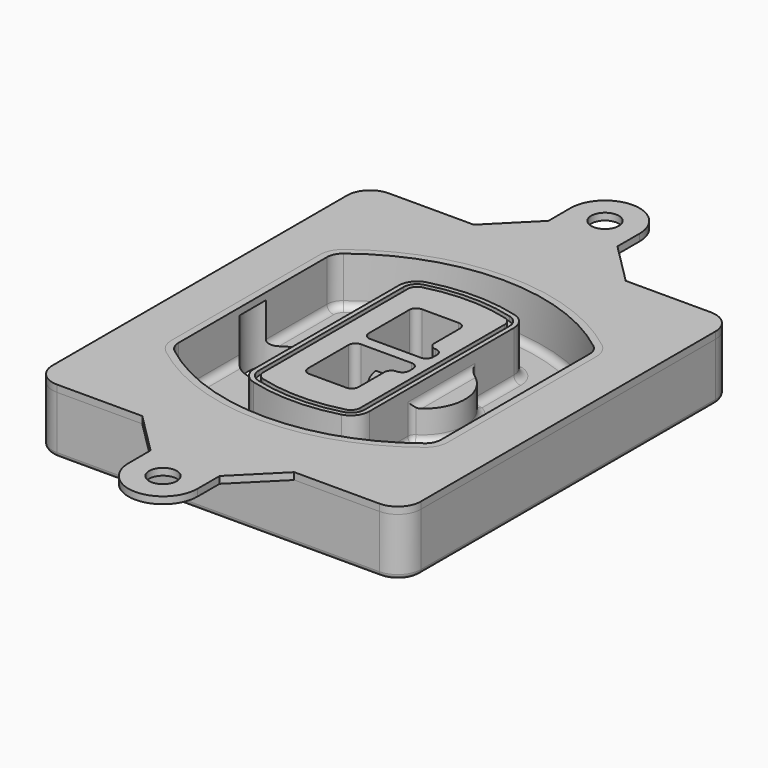
from build123d import *

# Parameters (mm, degrees)
F0_R      = 4
F1_DEPTH  = 25
F2_DEPTH  = 3
F3_DEPTH  = 18
F5_DEPTH  = 21
F6_DEPTH  = 2
F8_DEPTH  = 20
F9_DEPTH  = 16
F10_DEPTH = 25
F7_R      = 6
F7_R_2    = 4
F11_DEPTH = 6
F13_DEPTH = 9
F14_R     = 3
F16_R     = 2
F15_R     = 6
F17_DEPTH = 3


# Not quite as in the source:
# - a feature names something its author has since deleted; it is built from what else it names


with BuildPart() as f1:
    # F0 (on Top) → F1 (new body)
    with BuildSketch(Plane.XY):
        with BuildLine():
            ThreePointArc((-80, -80), (-77.0710678119, -87.0710678119), (-70, -90))
            Line((-70, -90), (70, -90))
            ThreePointArc((70, -90), (77.0710678119, -87.0710678119), (80, -80))
            Line((80, -80), (80, 80))
            ThreePointArc((80, 80), (77.0710678119, 87.0710678119), (70, 90))
            Line((70, 90), (-70, 90))
            ThreePointArc((-70, 90), (-77.0710678119, 87.0710678119), (-80, 80))
            Line((-80, 80), (-80, -80))
        make_face()
        with Locations((-60, -67.5)):
            Circle(F0_R, mode=Mode.SUBTRACT)
        with Locations((60, -67.5)):
            Circle(F0_R, mode=Mode.SUBTRACT)
        with Locations((-60, 67.5)):
            Circle(F0_R, mode=Mode.SUBTRACT)
        with BuildLine():
            ThreePointArc((-64, 40.2934422872), (-62.5820384798, 46.4328484224), (-58.6153846154, 51.3286200352))
            ThreePointArc((-58.6153846154, 51.3286200352), (0, 71.5), (58.6153846154, 51.3286200352))
            ThreePointArc((58.6153846154, 51.3286200352), (62.5820384798, 46.4328484224), (64, 40.2934422872))
            Line((64, 40.2934422872), (64, -40.2934422872))
            ThreePointArc((64, -40.2934422872), (62.5820384798, -46.4328484224), (58.6153846154, -51.3286200352))
            ThreePointArc((58.6153846154, -51.3286200352), (0, -71.5), (-58.6153846154, -51.3286200352))
            ThreePointArc((-58.6153846154, -51.3286200352), (-62.5820384798, -46.4328484224), (-64, -40.2934422872))
            Line((-64, -40.2934422872), (-64, 40.2934422872))
        make_face(mode=Mode.SUBTRACT)
        with Locations((60, 67.5)):
            Circle(F0_R, mode=Mode.SUBTRACT)
        with BuildLine():
            ThreePointArc((58.6153846154, 51.3286200352), (0, 71.5), (-58.6153846154, 51.3286200352))
            ThreePointArc((-58.6153846154, 51.3286200352), (-62.5820384798, 46.4328484224), (-64, 40.2934422872))
            Line((-64, 40.2934422872), (-64, -40.2934422872))
            ThreePointArc((-64, -40.2934422872), (-62.5820384798, -46.4328484224), (-58.6153846154, -51.3286200352))
            ThreePointArc((-58.6153846154, -51.3286200352), (0, -71.5), (58.6153846154, -51.3286200352))
            ThreePointArc((58.6153846154, -51.3286200352), (62.5820384798, -46.4328484224), (64, -40.2934422872))
            Line((64, -40.2934422872), (64, 40.2934422872))
            ThreePointArc((64, 40.2934422872), (62.5820384798, 46.4328484224), (58.6153846154, 51.3286200352))
        make_face()
        with BuildLine():
            Line((-60, -40.2934422872), (-60, 40.2934422872))
            ThreePointArc((-60, 40.2934422872), (-58.9871703427, 44.6787323838), (-56.1538461538, 48.1757121072))
            ThreePointArc((-56.1538461538, 48.1757121072), (0, 67.5), (56.1538461538, 48.1757121072))
            ThreePointArc((56.1538461538, 48.1757121072), (58.9871703427, 44.6787323838), (60, 40.2934422872))
            Line((60, 40.2934422872), (60, -40.2934422872))
            ThreePointArc((60, -40.2934422872), (58.9871703427, -44.6787323838), (56.1538461538, -48.1757121072))
            ThreePointArc((56.1538461538, -48.1757121072), (0, -67.5), (-56.1538461538, -48.1757121072))
            ThreePointArc((-56.1538461538, -48.1757121072), (-58.9871703427, -44.6787323838), (-60, -40.2934422872))
        make_face(mode=Mode.SUBTRACT)
        with BuildLine():
            ThreePointArc((-56.1538461538, 48.1757121072), (-58.9871703427, 44.6787323838), (-60, 40.2934422872))
            Line((-60, 40.2934422872), (-60, -40.2934422872))
            ThreePointArc((-60, -40.2934422872), (-58.9871703427, -44.6787323838), (-56.1538461538, -48.1757121072))
            ThreePointArc((-56.1538461538, -48.1757121072), (0, -67.5), (56.1538461538, -48.1757121072))
            ThreePointArc((56.1538461538, -48.1757121072), (58.9871703427, -44.6787323838), (60, -40.2934422872))
            Line((60, -40.2934422872), (60, 40.2934422872))
            ThreePointArc((60, 40.2934422872), (58.9871703427, 44.6787323838), (56.1538461538, 48.1757121072))
            ThreePointArc((56.1538461538, 48.1757121072), (0, 67.5), (-56.1538461538, 48.1757121072))
        make_face()
        with BuildLine():
            ThreePointArc((54.3076923077, 45.8110311612), (56.2910192399, 43.3631453548), (57, 40.2934422872))
            Line((57, 40.2934422872), (57, -40.2934422872))
            ThreePointArc((57, -40.2934422872), (56.2910192399, -43.3631453548), (54.3076923077, -45.8110311612))
            ThreePointArc((54.3076923077, -45.8110311612), (0, -64.5), (-54.3076923077, -45.8110311612))
            ThreePointArc((-54.3076923077, -45.8110311612), (-56.2910192399, -43.3631453548), (-57, -40.2934422872))
            Line((-57, -40.2934422872), (-57, 40.2934422872))
            ThreePointArc((-57, 40.2934422872), (-56.2910192399, 43.3631453548), (-54.3076923077, 45.8110311612))
            ThreePointArc((-54.3076923077, 45.8110311612), (0, 64.5), (54.3076923077, 45.8110311612))
        make_face(mode=Mode.SUBTRACT)
        with BuildLine():
            Line((57, -40.2934422872), (57, 40.2934422872))
            ThreePointArc((57, 40.2934422872), (56.2910192399, 43.3631453548), (54.3076923077, 45.8110311612))
            ThreePointArc((54.3076923077, 45.8110311612), (0, 64.5), (-54.3076923077, 45.8110311612))
            ThreePointArc((-54.3076923077, 45.8110311612), (-56.2910192399, 43.3631453548), (-57, 40.2934422872))
            Line((-57, 40.2934422872), (-57, -40.2934422872))
            ThreePointArc((-57, -40.2934422872), (-56.2910192399, -43.3631453548), (-54.3076923077, -45.8110311612))
            ThreePointArc((-54.3076923077, -45.8110311612), (0, -64.5), (54.3076923077, -45.8110311612))
            ThreePointArc((54.3076923077, -45.8110311612), (56.2910192399, -43.3631453548), (57, -40.2934422872))
        make_face()
    extrude(amount=-F1_DEPTH)

    # F0 (on Top) → F2 (join)
    with BuildSketch(Plane.XY):
        with BuildLine():
            ThreePointArc((-56.1538461538, 48.1757121072), (-58.9871703427, 44.6787323838), (-60, 40.2934422872))
            Line((-60, 40.2934422872), (-60, -40.2934422872))
            ThreePointArc((-60, -40.2934422872), (-58.9871703427, -44.6787323838), (-56.1538461538, -48.1757121072))
            ThreePointArc((-56.1538461538, -48.1757121072), (0, -67.5), (56.1538461538, -48.1757121072))
            ThreePointArc((56.1538461538, -48.1757121072), (58.9871703427, -44.6787323838), (60, -40.2934422872))
            Line((60, -40.2934422872), (60, 40.2934422872))
            ThreePointArc((60, 40.2934422872), (58.9871703427, 44.6787323838), (56.1538461538, 48.1757121072))
            ThreePointArc((56.1538461538, 48.1757121072), (0, 67.5), (-56.1538461538, 48.1757121072))
        make_face()
        with BuildLine():
            ThreePointArc((54.3076923077, 45.8110311612), (56.2910192399, 43.3631453548), (57, 40.2934422872))
            Line((57, 40.2934422872), (57, -40.2934422872))
            ThreePointArc((57, -40.2934422872), (56.2910192399, -43.3631453548), (54.3076923077, -45.8110311612))
            ThreePointArc((54.3076923077, -45.8110311612), (0, -64.5), (-54.3076923077, -45.8110311612))
            ThreePointArc((-54.3076923077, -45.8110311612), (-56.2910192399, -43.3631453548), (-57, -40.2934422872))
            Line((-57, -40.2934422872), (-57, 40.2934422872))
            ThreePointArc((-57, 40.2934422872), (-56.2910192399, 43.3631453548), (-54.3076923077, 45.8110311612))
            ThreePointArc((-54.3076923077, 45.8110311612), (0, 64.5), (54.3076923077, 45.8110311612))
        make_face(mode=Mode.SUBTRACT)
    extrude(amount=F2_DEPTH)

    # F0 (on Top) → F3 (cut)
    with BuildSketch(Plane.XY):
        with BuildLine():
            Line((57, -40.2934422872), (57, 40.2934422872))
            ThreePointArc((57, 40.2934422872), (56.2910192399, 43.3631453548), (54.3076923077, 45.8110311612))
            ThreePointArc((54.3076923077, 45.8110311612), (0, 64.5), (-54.3076923077, 45.8110311612))
            ThreePointArc((-54.3076923077, 45.8110311612), (-56.2910192399, 43.3631453548), (-57, 40.2934422872))
            Line((-57, 40.2934422872), (-57, -40.2934422872))
            ThreePointArc((-57, -40.2934422872), (-56.2910192399, -43.3631453548), (-54.3076923077, -45.8110311612))
            ThreePointArc((-54.3076923077, -45.8110311612), (0, -64.5), (54.3076923077, -45.8110311612))
            ThreePointArc((54.3076923077, -45.8110311612), (56.2910192399, -43.3631453548), (57, -40.2934422872))
        make_face()
    extrude(amount=-F3_DEPTH, mode=Mode.SUBTRACT)

    # F4 (on face) → F5 (join, through all)
    with BuildSketch(Plane.XY.offset(3)):
        with BuildLine():
            ThreePointArc((-25, -39.2465276821), (-23.3511545998, -44.1109737193), (-19.0842911877, -46.9702398883))
            ThreePointArc((-19.0842911877, -46.9702398883), (0, -49.5), (19.0842911877, -46.9702398883))
            ThreePointArc((19.0842911877, -46.9702398883), (23.3511545998, -44.1109737193), (25, -39.2465276821))
            Line((25, -39.2465276821), (25, 39.2465276821))
            ThreePointArc((25, 39.2465276821), (23.3511545998, 44.1109737193), (19.0842911877, 46.9702398883))
            ThreePointArc((19.0842911877, 46.9702398883), (0, 49.5), (-19.0842911877, 46.9702398883))
            ThreePointArc((-19.0842911877, 46.9702398883), (-23.3511545998, 44.1109737193), (-25, 39.2465276821))
            Line((-25, 39.2465276821), (-25, -39.2465276821))
        make_face()
        with BuildLine():
            ThreePointArc((18.5632183908, 45.0393118368), (21.7633659499, 42.89486221), (23, 39.2465276821))
            Line((23, 39.2465276821), (23, -39.2465276821))
            ThreePointArc((23, -39.2465276821), (21.7633659499, -42.89486221), (18.5632183908, -45.0393118368))
            ThreePointArc((18.5632183908, -45.0393118368), (0, -47.5), (-18.5632183908, -45.0393118368))
            ThreePointArc((-18.5632183908, -45.0393118368), (-21.7633659499, -42.89486221), (-23, -39.2465276821))
            Line((-23, -39.2465276821), (-23, 39.2465276821))
            ThreePointArc((-23, 39.2465276821), (-21.7633659499, 42.89486221), (-18.5632183908, 45.0393118368))
            ThreePointArc((-18.5632183908, 45.0393118368), (0, 47.5), (18.5632183908, 45.0393118368))
        make_face(mode=Mode.SUBTRACT)
        with BuildLine():
            Line((23, -39.2465276821), (23, 39.2465276821))
            ThreePointArc((23, 39.2465276821), (21.7633659499, 42.89486221), (18.5632183908, 45.0393118368))
            ThreePointArc((18.5632183908, 45.0393118368), (0, 47.5), (-18.5632183908, 45.0393118368))
            ThreePointArc((-18.5632183908, 45.0393118368), (-21.7633659499, 42.89486221), (-23, 39.2465276821))
            Line((-23, 39.2465276821), (-23, -39.2465276821))
            ThreePointArc((-23, -39.2465276821), (-21.7633659499, -42.89486221), (-18.5632183908, -45.0393118368))
            ThreePointArc((-18.5632183908, -45.0393118368), (0, -47.5), (18.5632183908, -45.0393118368))
            ThreePointArc((18.5632183908, -45.0393118368), (21.7633659499, -42.89486221), (23, -39.2465276821))
        make_face()
        with BuildLine():
            ThreePointArc((18.0421455939, 43.1083837852), (20.1755772999, 41.6787507007), (21, 39.2465276821))
            Line((21, 39.2465276821), (21, -39.2465276821))
            ThreePointArc((21, -39.2465276821), (20.1755772999, -41.6787507007), (18.0421455939, -43.1083837852))
            ThreePointArc((18.0421455939, -43.1083837852), (0, -45.5), (-18.0421455939, -43.1083837852))
            ThreePointArc((-18.0421455939, -43.1083837852), (-20.1755772999, -41.6787507007), (-21, -39.2465276821))
            Line((-21, -39.2465276821), (-21, 39.2465276821))
            ThreePointArc((-21, 39.2465276821), (-20.1755772999, 41.6787507007), (-18.0421455939, 43.1083837852))
            ThreePointArc((-18.0421455939, 43.1083837852), (0, 45.5), (18.0421455939, 43.1083837852))
        make_face(mode=Mode.SUBTRACT)
        with BuildLine():
            Line((21, -39.2465276821), (21, 39.2465276821))
            ThreePointArc((21, 39.2465276821), (20.1755772999, 41.6787507007), (18.0421455939, 43.1083837852))
            ThreePointArc((18.0421455939, 43.1083837852), (0, 45.5), (-18.0421455939, 43.1083837852))
            ThreePointArc((-18.0421455939, 43.1083837852), (-20.1755772999, 41.6787507007), (-21, 39.2465276821))
            Line((-21, 39.2465276821), (-21, -39.2465276821))
            ThreePointArc((-21, -39.2465276821), (-20.1755772999, -41.6787507007), (-18.0421455939, -43.1083837852))
            ThreePointArc((-18.0421455939, -43.1083837852), (0, -45.5), (18.0421455939, -43.1083837852))
            ThreePointArc((18.0421455939, -43.1083837852), (20.1755772999, -41.6787507007), (21, -39.2465276821))
        make_face()
        with BuildLine():
            Line((-8, -2.5), (14, -2.5))
            ThreePointArc((14, -2.5), (16.1213203436, -3.3786796564), (17, -5.5))
            Line((17, -5.5), (17, -7.5))
            ThreePointArc((17, -7.5), (16.1213203436, -9.6213203436), (14, -10.5))
            ThreePointArc((14, -10.5), (11.8786796564, -11.3786796564), (11, -13.5))
            Line((11, -13.5), (11, -27.5))
            ThreePointArc((11, -27.5), (10.1213203436, -29.6213203436), (8, -30.5))
            Line((8, -30.5), (-8, -30.5))
            ThreePointArc((-8, -30.5), (-10.1213203436, -29.6213203436), (-11, -27.5))
            Line((-11, -27.5), (-11, -5.5))
            ThreePointArc((-11, -5.5), (-10.1213203436, -3.3786796564), (-8, -2.5))
        make_face(mode=Mode.SUBTRACT)
        with BuildLine():
            ThreePointArc((-8, 2.5), (-10.1213203436, 3.3786796564), (-11, 5.5))
            Line((-11, 5.5), (-11, 27.5))
            ThreePointArc((-11, 27.5), (-10.1213203436, 29.6213203436), (-8, 30.5))
            Line((-8, 30.5), (8, 30.5))
            ThreePointArc((8, 30.5), (10.1213203436, 29.6213203436), (11, 27.5))
            Line((11, 27.5), (11, 13.5))
            ThreePointArc((11, 13.5), (11.8786796564, 11.3786796564), (14, 10.5))
            ThreePointArc((14, 10.5), (16.1213203436, 9.6213203436), (17, 7.5))
            Line((17, 7.5), (17, 5.5))
            ThreePointArc((17, 5.5), (16.1213203436, 3.3786796564), (14, 2.5))
            Line((14, 2.5), (-8, 2.5))
        make_face(mode=Mode.SUBTRACT)
    extrude(amount=-F5_DEPTH)

    # F4 (on face) → F6 (cut)
    with BuildSketch(Plane.XY.offset(3)):
        with BuildLine():
            Line((23, -39.2465276821), (23, 39.2465276821))
            ThreePointArc((23, 39.2465276821), (21.7633659499, 42.89486221), (18.5632183908, 45.0393118368))
            ThreePointArc((18.5632183908, 45.0393118368), (0, 47.5), (-18.5632183908, 45.0393118368))
            ThreePointArc((-18.5632183908, 45.0393118368), (-21.7633659499, 42.89486221), (-23, 39.2465276821))
            Line((-23, 39.2465276821), (-23, -39.2465276821))
            ThreePointArc((-23, -39.2465276821), (-21.7633659499, -42.89486221), (-18.5632183908, -45.0393118368))
            ThreePointArc((-18.5632183908, -45.0393118368), (0, -47.5), (18.5632183908, -45.0393118368))
            ThreePointArc((18.5632183908, -45.0393118368), (21.7633659499, -42.89486221), (23, -39.2465276821))
        make_face()
        with BuildLine():
            ThreePointArc((18.0421455939, 43.1083837852), (20.1755772999, 41.6787507007), (21, 39.2465276821))
            Line((21, 39.2465276821), (21, -39.2465276821))
            ThreePointArc((21, -39.2465276821), (20.1755772999, -41.6787507007), (18.0421455939, -43.1083837852))
            ThreePointArc((18.0421455939, -43.1083837852), (0, -45.5), (-18.0421455939, -43.1083837852))
            ThreePointArc((-18.0421455939, -43.1083837852), (-20.1755772999, -41.6787507007), (-21, -39.2465276821))
            Line((-21, -39.2465276821), (-21, 39.2465276821))
            ThreePointArc((-21, 39.2465276821), (-20.1755772999, 41.6787507007), (-18.0421455939, 43.1083837852))
            ThreePointArc((-18.0421455939, 43.1083837852), (0, 45.5), (18.0421455939, 43.1083837852))
        make_face(mode=Mode.SUBTRACT)
    extrude(amount=-F6_DEPTH, mode=Mode.SUBTRACT)

    # F7 (on face) → F8 (join)
    with BuildSketch(Plane(origin=(0, 0, -25), x_dir=(1, 0, 0), z_dir=(0, 0, -1))):
        with BuildLine():
            ThreePointArc((3.28842436, 0), (16.7567035675, 13.4682792075), (30.224982775, 0))
            Line((30.224982775, 0), (35.224982775, 0))
            ThreePointArc((35.224982775, 0), (16.7567035675, 18.4682792075), (-1.71157564, 0))
            Line((-1.71157564, 0), (3.28842436, 0))
        make_face()
        with BuildLine():
            Line((3.28842436, 0), (30.224982775, 0))
            ThreePointArc((30.224982775, 0), (16.7567035675, 13.4682792075), (3.28842436, 0))
        make_face()
        with BuildLine():
            ThreePointArc((3.28842436, 0), (16.7567035675, -13.4682792075), (30.224982775, 0))
            Line((30.224982775, 0), (3.28842436, 0))
        make_face()
        with BuildLine():
            Line((35.224982775, 0), (30.224982775, 0))
            ThreePointArc((30.224982775, 0), (16.7567035675, -13.4682792075), (3.28842436, 0))
            Line((3.28842436, 0), (-1.71157564, 0))
            ThreePointArc((-1.71157564, 0), (16.7567035675, -18.4682792075), (35.224982775, 0))
        make_face()
    extrude(amount=-F8_DEPTH)

    # F7 (on face) → F9 (cut)
    with BuildSketch(Plane(origin=(0, 0, -25), x_dir=(1, 0, 0), z_dir=(0, 0, -1))):
        with BuildLine():
            Line((3.28842436, 0), (30.224982775, 0))
            ThreePointArc((30.224982775, 0), (16.7567035675, 13.4682792075), (3.28842436, 0))
        make_face()
        with BuildLine():
            ThreePointArc((3.28842436, 0), (16.7567035675, -13.4682792075), (30.224982775, 0))
            Line((30.224982775, 0), (3.28842436, 0))
        make_face()
    extrude(amount=-F9_DEPTH, mode=Mode.SUBTRACT)

    # F7 (on face) → F10 (cut)
    with BuildSketch(Plane(origin=(0, 0, -25), x_dir=(1, 0, 0), z_dir=(0, 0, -1))):
        with BuildLine():
            Line((-59.0318229325, 0), (-32.0952645175, 0))
            ThreePointArc((-32.0952645175, 0), (-45.563543725, 13.4682792075), (-59.0318229325, 0))
        make_face()
        with BuildLine():
            ThreePointArc((-59.0318229325, 0), (-45.563543725, -13.4682792075), (-32.0952645175, 0))
            Line((-32.0952645175, 0), (-59.0318229325, 0))
        make_face()
    extrude(amount=-F10_DEPTH, mode=Mode.SUBTRACT)

    # F7 (on face) → F11 (cut)
    with BuildSketch(Plane(origin=(0, 0, -25), x_dir=(1, 0, 0), z_dir=(0, 0, -1))):
        with Locations((60, -67.5)):
            Circle(F7_R)
        with Locations((60, -67.5)):
            Circle(F7_R_2, mode=Mode.SUBTRACT)
        with Locations((-60, -67.5)):
            Circle(F7_R)
        with Locations((-60, -67.5)):
            Circle(F7_R_2, mode=Mode.SUBTRACT)
        with Locations((-60, 67.5)):
            Circle(F7_R)
        with Locations((-60, 67.5)):
            Circle(F7_R_2, mode=Mode.SUBTRACT)
        with Locations((60, 67.5)):
            Circle(F7_R)
        with Locations((60, 67.5)):
            Circle(F7_R_2, mode=Mode.SUBTRACT)
    extrude(amount=-F11_DEPTH, mode=Mode.SUBTRACT)

    # F12 (on face) → F13 (cut, through all)
    with BuildSketch(Plane(origin=(0, 0, -9), x_dir=(1, 0, 0), z_dir=(0, 0, -1))):
        with BuildLine():
            Line((11, 13.5), (11, 17.5481537753))
            ThreePointArc((11, 17.5481537753), (2.5696536419, 11.8239143813), (-1.5415842455, 2.5))
            Line((-1.5415842455, 2.5), (3.5224848595, 2.5))
            ThreePointArc((3.5224848595, 2.5), (6.1857188154, 8.3455872281), (11.2536447004, 12.2927168648))
            ThreePointArc((11.2536447004, 12.2927168648), (11.0640958889, 12.8831798879), (11, 13.5))
        make_face()
        with BuildLine():
            ThreePointArc((11.2536447004, -12.2927168648), (6.1857188154, -8.3455872281), (3.5224848595, -2.5))
            Line((3.5224848595, -2.5), (-1.5415842455, -2.5))
            ThreePointArc((-1.5415842455, -2.5), (2.5696536419, -11.8239143813), (11, -17.5481537753))
            Line((11, -17.5481537753), (11, -13.5))
            ThreePointArc((11, -13.5), (11.0640958889, -12.8831798879), (11.2536447004, -12.2927168648))
        make_face()
        with BuildLine():
            ThreePointArc((11.2536447004, 12.2927168648), (6.1857188154, 8.3455872281), (3.5224848595, 2.5))
            Line((3.5224848595, 2.5), (14, 2.5))
            ThreePointArc((14, 2.5), (16.1213203436, 3.3786796564), (17, 5.5))
            Line((17, 5.5), (17, 7.5))
            ThreePointArc((17, 7.5), (16.1213203436, 9.6213203436), (14, 10.5))
            ThreePointArc((14, 10.5), (12.3601599782, 10.9878446101), (11.2536447004, 12.2927168648))
        make_face()
        with BuildLine():
            Line((14, -2.5), (3.5224848595, -2.5))
            ThreePointArc((3.5224848595, -2.5), (6.1857188154, -8.3455872281), (11.2536447004, -12.2927168648))
            ThreePointArc((11.2536447004, -12.2927168648), (12.3601599782, -10.9878446101), (14, -10.5))
            ThreePointArc((14, -10.5), (16.1213203436, -9.6213203436), (17, -7.5))
            Line((17, -7.5), (17, -5.5))
            ThreePointArc((17, -5.5), (16.1213203436, -3.3786796564), (14, -2.5))
        make_face()
    extrude(amount=F13_DEPTH, mode=Mode.SUBTRACT)

    # F14
    f14_edges = [f1.edges().sort_by_distance(p)[0] for p in [
        (-57, -23.703476, -18),
        (-57, 23.703476, -18),
        (25, 0, -5),
        (25, 16.526506, -11.5),
        (25, -16.526506, -11.5),
        (25, -27.886517, -18),
        (35.224983, 0, -18),
    ]]
    fillet(f14_edges, radius=F14_R)

    # F16
    f16_edges = [f1.edges().sort_by_distance(p)[0] for p in [
        (0, -90, -25),
    ]]
    fillet(f16_edges, radius=F16_R)


with BuildPart() as f17:
    # F15 (on Top) → F17 (new body, through all)
    with BuildSketch(Plane.XY):
        with BuildLine():
            Line((-15, 108), (-33, 90))
            Line((-33, 90), (33, 90))
            Line((33, 90), (15, 108))
            Line((15, 108), (15, 120))
            ThreePointArc((15, 120), (0, 135), (-15, 120))
            Line((-15, 120), (-15, 108))
        make_face()
        with Locations((0, 120)):
            Circle(F15_R, mode=Mode.SUBTRACT)
        with BuildLine():
            Line((33, -90), (-33, -90))
            Line((-33, -90), (-15, -108))
            Line((-15, -108), (-15, -120))
            ThreePointArc((-15, -120), (0, -135), (15, -120))
            Line((15, -120), (15, -108))
            Line((15, -108), (33, -90))
        make_face()
        with Locations((0, -120)):
            Circle(F15_R, mode=Mode.SUBTRACT)
        with BuildLine():
            Line((-33, 90), (-70, 90))
            ThreePointArc((-70, 90), (-77.0710678119, 87.0710678119), (-80, 80))
            Line((-80, 80), (-80, -80))
            ThreePointArc((-80, -80), (-77.0710678119, -87.0710678119), (-70, -90))
            Line((-70, -90), (-33, -90))
            Line((-33, -90), (33, -90))
            Line((33, -90), (70, -90))
            ThreePointArc((70, -90), (77.0710678119, -87.0710678119), (80, -80))
            Line((80, -80), (80, 80))
            ThreePointArc((80, 80), (77.0710678119, 87.0710678119), (70, 90))
            Line((70, 90), (33, 90))
            Line((33, 90), (-33, 90))
        make_face()
        with BuildLine():
            ThreePointArc((-56.1538461538, 48.1757121072), (0, 67.5), (56.1538461538, 48.1757121072))
            ThreePointArc((56.1538461538, 48.1757121072), (58.9871703427, 44.6787323838), (60, 40.2934422872))
            Line((60, 40.2934422872), (60, -40.2934422872))
            ThreePointArc((60, -40.2934422872), (58.9871703427, -44.6787323838), (56.1538461538, -48.1757121072))
            ThreePointArc((56.1538461538, -48.1757121072), (0, -67.5), (-56.1538461538, -48.1757121072))
            ThreePointArc((-56.1538461538, -48.1757121072), (-58.9871703427, -44.6787323838), (-60, -40.2934422872))
            Line((-60, -40.2934422872), (-60, 40.2934422872))
            ThreePointArc((-60, 40.2934422872), (-58.9871703427, 44.6787323838), (-56.1538461538, 48.1757121072))
        make_face(mode=Mode.SUBTRACT)
    extrude(amount=F17_DEPTH)


solid = Compound([f1.part, f17.part])
